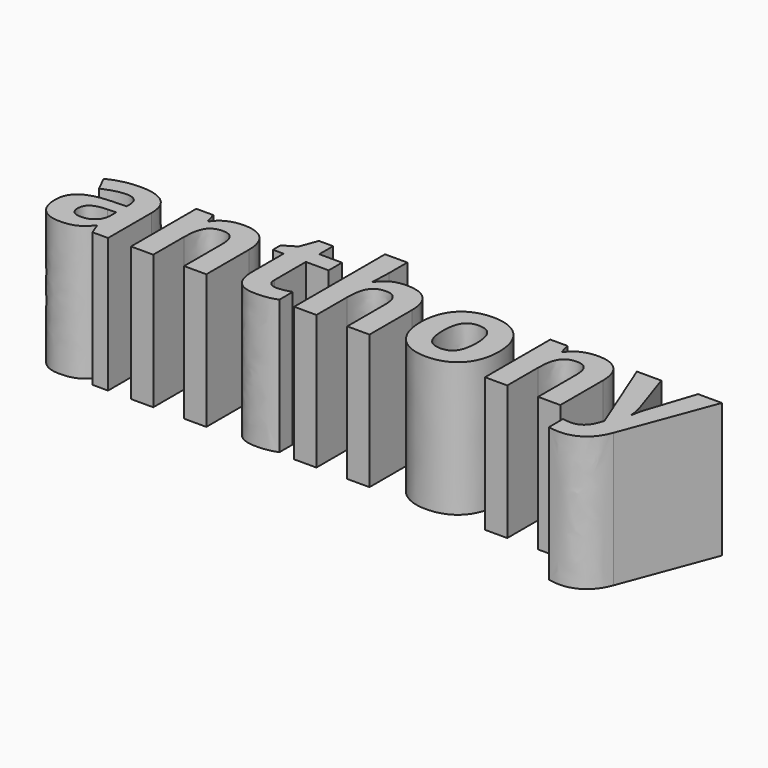
from build123d import *

# Parameters (mm, degrees)
F0_TEXT_SIZE = 84.7954794558
F1_DEPTH     = 76.2


# Not quite as in the source:
# - Text() gives the source's letters only with a copy of the font that has no kerning and outlines rounded to 1/6400 em; it was checked with that copy


with BuildPart() as f1:
    # F0 (on Top) → F1 (new body)
    with BuildSketch(Plane.XY):
        with Locations((-157.4631021358, -28.9575066417)):
            Text('anthony', F0_TEXT_SIZE, font='Open Sans', font_style=FontStyle.BOLD, text_align=(TextAlign.LEFT, TextAlign.BOTTOM))
    extrude(amount=F1_DEPTH)


solid = f1.part
